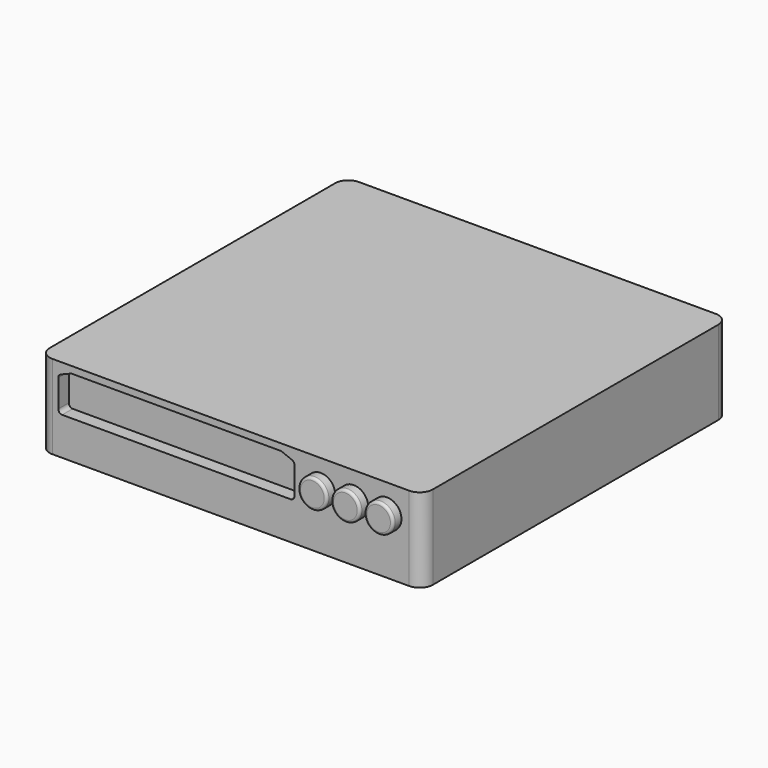
from build123d import *

# Parameters (mm, degrees)
F1_DEPTH    = 32
F2_R        = 5.5
F3_DEPTH    = 4
F4_R        = 1
F2_W        = 90
F2_H        = 15
F5_DEPTH    = 5
F6_T1_DEPTH = 17.9655681957
F7_SIZE2    = 2
F7_SIZE     = 5
F8_R        = 1.5
F9_R        = 6.3934301863
F9_R_2      = 6.243428201
F10_DEPTH   = 15


# Not quite as in the source:
# - a fillet or chamfer that OpenCascade refuses, or shapes differently, is made with other operations: its cross-section is extruded or revolved along the edge and cut away or added


with BuildPart() as f1:
    # F0 (on Top) → F1 (new body)
    with BuildSketch(Plane.XY):
        with BuildLine():
            ThreePointArc((0, 5), (1.4644660941, 1.4644660941), (5, 0))
            Line((5, 0), (141, 0))
            ThreePointArc((141, 0), (144.5355339059, 1.4644660941), (146, 5))
            Line((146, 5), (146, 141))
            ThreePointArc((146, 141), (144.5355339059, 144.5355339059), (141, 146))
            Line((141, 146), (5, 146))
            ThreePointArc((5, 146), (1.4644660941, 144.5355339059), (0, 141))
            Line((0, 141), (0, 5))
        make_face()
    extrude(amount=F1_DEPTH)

    # F2 (on face) → F3 (join)
    with BuildSketch(Plane.XZ):
        with Locations((107.308909297, 21.5077847242)):
            Circle(F2_R)
        with Locations((119.8735386133, 21.5077847242)):
            Circle(F2_R)
        with Locations((132.552921772, 21.5077847242)):
            Circle(F2_R)
    extrude(amount=F3_DEPTH)

    # F4
    f4_edges = [f1.edges().sort_by_distance(p)[0] for p in [
        (101.808909, -4, 21.507785),
        (114.373539, -4, 21.507785),
        (127.052922, -4, 21.507785),
    ]]
    fillet(f4_edges, radius=F4_R)

    # F2 (on face) → F5 (cut)
    with BuildSketch(Plane.XZ):
        with Locations((52.2508216836, 21.9252242893)):
            Rectangle(F2_W, F2_H)
    extrude(amount=-F5_DEPTH, mode=Mode.SUBTRACT)

    # F6: chamfer of 2 x 5 on 1 edges, made by hand

    # F6_s2 → F6_t1 (join)
    with BuildSketch(Plane.XZ.offset(-17.9655681957)):
        Polygon((12.2508216836, 29.4252242893), (7.2508216836, 27.4252242893), (7.2508216836, 29.4252242893), align=None)
    extrude(amount=F6_T1_DEPTH)

    # F7
    f7_edges = [f1.edges().sort_by_distance(p)[0] for p in [
        (97.250822, 2.5, 29.425224),
    ]]
    chamfer(f7_edges, length=F7_SIZE, length2=F7_SIZE2)

    # F8
    f8_edges = [f1.edges().sort_by_distance(p)[0] for p in [
        (92.250822, 2.5, 29.425224),
        (97.250822, 2.5, 27.425224),
        (97.250822, 2.5, 14.425224),
        (7.250822, 2.5, 14.425224),
        (7.250822, 2.5, 27.425224),
        (12.250822, 2.5, 29.425224),
    ]]
    fillet(f8_edges, radius=F8_R)

    # F9 (on face) → F10 (join)
    with BuildSketch(Plane(origin=(0, 146, 0), x_dir=(-1, 0, 0), z_dir=(0, 1, 0))):
        with Locations((-90.0897681713, 13.0425486714)):
            Circle(F9_R)
        with Locations((-69.4026425481, 13.0425486714)):
            Circle(F9_R_2)
    extrude(amount=F10_DEPTH)


solid = f1.part
